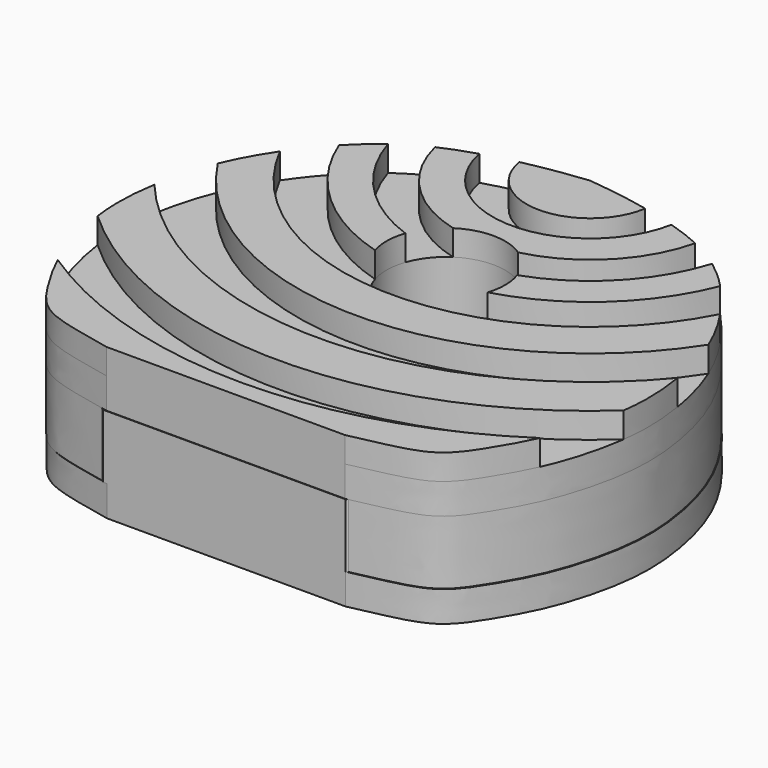
from build123d import *

# Parameters (mm, degrees)
F1_DEPTH  = 2.5
F2_R      = 2.2928226191
F3_DEPTH  = 25.4
F5_DEPTH  = 1.2
F8_DEPTH  = 2.5
F9_DEPTH  = 1.2
F10_R     = 2.3288193764
F11_DEPTH = 25.4
F13_DEPTH = 1


# Not quite as in the source:
# - after a boolean that leaves OpenCascade's solid faulty, fix() repairs it


with BuildPart() as f1:
    # F0 (on Top) → F1 (new body)
    with BuildSketch(Plane.XY):
        with BuildLine():
            ThreePointArc((-8.9879343286, 39.4452884793), (-13.7471402995, 56.3640609225), (-18.5063462704, 39.4452884793))
            Line((-18.5063462704, 39.4452884793), (-8.9879343286, 39.4452884793))
        make_face()
    extrude(amount=F1_DEPTH)

    # F2 (on Top) → F3 (cut)
    with BuildSketch(Plane.XY):
        with Locations((-13.6671839282, 50.2410940826)):
            Circle(F2_R)
    extrude(amount=F3_DEPTH, mode=Mode.SUBTRACT)

    # F4 (on Top) → F5 (join)
    with BuildSketch(Plane.XY):
        with BuildLine():
            add(Edge.make_bspline(
                [(-13.6700998992, 57.3167428374), (-12.2791459013, 57.1776458416), (-9.0720580617, 56.5741155476), (-6.3520616613, 54.8008037838), (-4.1044958722, 51.7145145132), (-3.3277388361, 48.8343071743), (-3.1695344368, 46.2953832393), (-3.9427728458, 43.353155853), (-4.9861142684, 41.5734784894), (-6.0248466508, 39.9837351848), (-7.6451300521, 39.7473392392), (-8.9879343286, 39.4452884793)],
                knots=[0, 0, 0, 0, 0.1391131435, 0.256793187, 0.3818563281, 0.493472527, 0.5970664143, 0.7096475295, 0.8035052556, 0.8866680838, 1, 1, 1, 1], degree=3))
            add(Edge.make_bspline(
                [(-13.6700998992, 57.3167428374), (-15.061053897, 57.1776458416), (-18.2681417367, 56.5741155476), (-20.988138137, 54.8008037838), (-23.2357039261, 51.7145145132), (-24.0124609622, 48.8343071743), (-24.1706653616, 46.2953832393), (-23.3974269525, 43.353155853), (-22.35408553, 41.5734784894), (-21.3153531475, 39.9837351848), (-19.6950697463, 39.7473392392), (-18.3522654697, 39.4452884793)],
                knots=[0, 0, 0, 0, 0.1391131435, 0.256793187, 0.3818563281, 0.493472527, 0.5970664143, 0.7096475295, 0.8035052556, 0.8866680838, 1, 1, 1, 1], degree=3))
            Line((-18.3522654697, 39.4452884793), (-8.9879343286, 39.4452884793))
        make_face()
    extrude(amount=-F5_DEPTH)

    # F7 (on offset) → F8 (join)
    with BuildSketch(Plane.XY.offset(2.5)):
        with BuildLine():
            add(Edge.make_bspline(
                [(-13.7050435878, 57.337269187), (-12.31408959, 57.1981721911), (-9.1070017503, 56.5946418971), (-6.38700535, 54.8213301333), (-4.1394395609, 51.7350408627), (-3.3626825248, 48.8548335238), (-3.2044781254, 46.3159095888), (-3.9777165345, 43.3736822025), (-5.021057957, 41.594004839), (-6.0597903395, 40.0042615343), (-7.6800737407, 39.7678655887), (-9.0228780173, 39.4658148289)],
                knots=[0, 0, 0, 0, 0.1391131435, 0.256793187, 0.3818563281, 0.493472527, 0.5970664143, 0.7096475295, 0.8035052556, 0.8866680838, 1, 1, 1, 1], degree=3))
            add(Edge.make_bspline(
                [(-13.7050435878, 57.337269187), (-15.0959975857, 57.1981721911), (-18.3030854253, 56.5946418971), (-21.0230818257, 54.8213301333), (-23.2706476148, 51.7350408627), (-24.0474046509, 48.8548335238), (-24.2056090503, 46.3159095888), (-23.4323706412, 43.3736822025), (-22.3890292186, 41.594004839), (-21.3502968362, 40.0042615343), (-19.7300134349, 39.7678655887), (-18.3872091584, 39.4658148289)],
                knots=[0, 0, 0, 0, 0.1391131435, 0.256793187, 0.3818563281, 0.493472527, 0.5970664143, 0.7096475295, 0.8035052556, 0.8866680838, 1, 1, 1, 1], degree=3))
            Line((-18.3872091584, 39.4658148289), (-9.0228780173, 39.4658148289))
        make_face()
    extrude(amount=-F8_DEPTH)

    # F7 (on offset) → F9 (join)
    with BuildSketch(Plane.XY.offset(2.5)):
        with BuildLine():
            add(Edge.make_bspline(
                [(-13.7050435878, 57.337269187), (-12.31408959, 57.1981721911), (-9.1070017503, 56.5946418971), (-6.38700535, 54.8213301333), (-4.1394395609, 51.7350408627), (-3.3626825248, 48.8548335238), (-3.2044781254, 46.3159095888), (-3.9777165345, 43.3736822025), (-5.021057957, 41.594004839), (-6.0597903395, 40.0042615343), (-7.6800737407, 39.7678655887), (-9.0228780173, 39.4658148289)],
                knots=[0, 0, 0, 0, 0.1391131435, 0.256793187, 0.3818563281, 0.493472527, 0.5970664143, 0.7096475295, 0.8035052556, 0.8866680838, 1, 1, 1, 1], degree=3))
            add(Edge.make_bspline(
                [(-13.7050435878, 57.337269187), (-15.0959975857, 57.1981721911), (-18.3030854253, 56.5946418971), (-21.0230818257, 54.8213301333), (-23.2706476148, 51.7350408627), (-24.0474046509, 48.8548335238), (-24.2056090503, 46.3159095888), (-23.4323706412, 43.3736822025), (-22.3890292186, 41.594004839), (-21.3502968362, 40.0042615343), (-19.7300134349, 39.7678655887), (-18.3872091584, 39.4658148289)],
                knots=[0, 0, 0, 0, 0.1391131435, 0.256793187, 0.3818563281, 0.493472527, 0.5970664143, 0.7096475295, 0.8035052556, 0.8866680838, 1, 1, 1, 1], degree=3))
            Line((-18.3872091584, 39.4658148289), (-9.0228780173, 39.4658148289))
        make_face()
    extrude(amount=F9_DEPTH)

    # F10 (on face) → F11 (cut)
    with BuildSketch(Plane.XY.offset(3.7)):
        with Locations((-13.7454718351, 50.3010265529)):
            Circle(F10_R)
    extrude(amount=-F11_DEPTH, mode=Mode.SUBTRACT)

    # F12 (on face) → F13 (join)
    with BuildSketch(Plane.XY.offset(3.7)):
        with BuildLine():
            add(Edge.make_bspline(
                [(-13.7050435878, 57.337269187), (-14.4653313277, 57.2612395406), (-15.3291200458, 57.1290853585), (-16.1737990809, 56.9432560968)],
                knots=[0, 0, 0, 0, 0.0760384726, 0.0760384726, 0.0760384726, 0.0760384726], degree=3))
            ThreePointArc((-16.1737990809, 56.9432560968), (-13.7050435878, 54.837269187), (-11.2362880947, 56.9432560968))
            add(Edge.make_bspline(
                [(-13.7050435878, 57.337269187), (-12.944755848, 57.2612395406), (-12.0809671299, 57.1290853585), (-11.2362880947, 56.9432560968)],
                knots=[0, 0, 0, 0, 0.0760384726, 0.0760384726, 0.0760384726, 0.0760384726], degree=3))
        make_face()
        with BuildLine():
            ThreePointArc((-9.9368932211, 56.6057620793), (-13.7050435878, 53.4987721067), (-17.4731939546, 56.6057620793))
            add(Edge.make_bspline(
                [(-17.4731939546, 56.6057620793), (-17.713095027, 56.5324460832), (-18.1815017641, 56.3748215542), (-18.6046452919, 56.1978491764), (-18.8084564971, 56.1028285931)],
                knots=[0.1160410133, 0.1160410133, 0.1160410133, 0.1160410133, 0.1391131435, 0.1625827971, 0.1625827971, 0.1625827971, 0.1625827971], degree=3))
            ThreePointArc((-18.8084564971, 56.1028285931), (-17.4454527537, 53.6524345673), (-15.0157350202, 52.2529054243))
            ThreePointArc((-15.0157350202, 52.2529054243), (-13.7320913228, 52.6298074893), (-12.452863378, 52.2381798934))
            ThreePointArc((-12.452863378, 52.2381798934), (-9.9858678234, 53.6310044183), (-8.6016306786, 56.1028285931))
            add(Edge.make_bspline(
                [(-9.9368932211, 56.6057620793), (-9.6969921487, 56.5324460832), (-9.2285854116, 56.3748215542), (-8.8054418837, 56.1978491764), (-8.6016306786, 56.1028285931)],
                knots=[0.1160410133, 0.1160410133, 0.1160410133, 0.1160410133, 0.1391131435, 0.1625827971, 0.1625827971, 0.1625827971, 0.1625827971], degree=3))
        make_face()
        with BuildLine():
            ThreePointArc((-15.9439411579, 51.0692272588), (-18.5092523241, 52.7306879861), (-20.0615521842, 55.3634884478))
            add(Edge.make_bspline(
                [(-20.0615521842, 55.3634884478), (-20.3622908826, 55.1424226516), (-20.7354717832, 54.8211081374), (-21.0991869423, 54.4504855004), (-21.184759468, 54.3600266085)],
                knots=[0.2154149552, 0.2154149552, 0.2154149552, 0.2154149552, 0.256793187, 0.2696740176, 0.2696740176, 0.2696740176, 0.2696740176], degree=3))
            ThreePointArc((-21.184759468, 54.3600266085), (-19.1249825347, 51.3845903924), (-15.9700219432, 49.6119862751))
            ThreePointArc((-15.9700219432, 49.6119862751), (-16.0739183221, 50.342699628), (-15.9439411579, 51.0692272588))
        make_face()
        with BuildLine():
            add(Edge.make_bspline(
                [(-7.3485349914, 55.3634884478), (-7.0477962931, 55.1424226516), (-6.6746153925, 54.8211081374), (-6.3109002333, 54.4504855004), (-6.2253277077, 54.3600266085)],
                knots=[0.2154149552, 0.2154149552, 0.2154149552, 0.2154149552, 0.256793187, 0.2696740176, 0.2696740176, 0.2696740176, 0.2696740176], degree=3))
            ThreePointArc((-7.3485349914, 55.3634884478), (-8.9273818183, 52.703160863), (-11.538320231, 51.0439138151))
            ThreePointArc((-11.538320231, 51.0439138151), (-11.4472706788, 50.6774188121), (-11.4166524587, 50.3010265529))
            ThreePointArc((-11.4166524587, 50.3010265529), (-11.4449073479, 49.9393599552), (-11.5289863986, 49.586469349))
            ThreePointArc((-11.5289863986, 49.586469349), (-8.319395937, 51.3535477363), (-6.2253277077, 54.3600266085))
        make_face()
        with BuildLine():
            ThreePointArc((-5.0678640605, 52.9127318674), (-13.7050435878, 47.632765043), (-22.3422231152, 52.9127318674))
            add(Edge.make_bspline(
                [(-22.3422231152, 52.9127318674), (-22.6243676708, 52.4958290759), (-22.9828123106, 51.88389324), (-23.2550467817, 51.2771618886), (-23.3282983496, 51.0995423986)],
                knots=[0.3317914228, 0.3317914228, 0.3317914228, 0.3317914228, 0.3818563281, 0.4026844082, 0.4026844082, 0.4026844082, 0.4026844082], degree=3))
            ThreePointArc((-23.3282983496, 51.0995423986), (-13.7050435878, 45.8692149625), (-4.0817888261, 51.0995423986))
            add(Edge.make_bspline(
                [(-5.0678640605, 52.9127318674), (-4.7857195048, 52.4958290759), (-4.427274865, 51.88389324), (-4.155040394, 51.2771618886), (-4.0817888261, 51.0995423986)],
                knots=[0.3317914228, 0.3317914228, 0.3317914228, 0.3317914228, 0.3818563281, 0.4026844082, 0.4026844082, 0.4026844082, 0.4026844082], degree=3))
        make_face()
        with BuildLine():
            ThreePointArc((-3.442200784, 48.7899550221), (-13.7050435878, 43.9812772041), (-23.9678863916, 48.7899550221))
            add(Edge.make_bspline(
                [(-23.9678863916, 48.7899550221), (-24.1027753964, 47.9656433641), (-24.1537367431, 47.107497335), (-24.0362338424, 46.1506221844), (-24.0261197487, 46.0757155585)],
                knots=[0.4950631574, 0.4950631574, 0.4950631574, 0.4950631574, 0.5970664143, 0.6056719545, 0.6056719545, 0.6056719545, 0.6056719545], degree=3))
            ThreePointArc((-24.0261197487, 46.0757155585), (-13.7050435878, 42.0615628777), (-3.3839674269, 46.0757155585))
            add(Edge.make_bspline(
                [(-3.442200784, 48.7899550221), (-3.3073117793, 47.9656433641), (-3.2563504326, 47.107497335), (-3.3738533332, 46.1506221844), (-3.3839674269, 46.0757155585)],
                knots=[0.4950631574, 0.4950631574, 0.4950631574, 0.4950631574, 0.5970664143, 0.6056719545, 0.6056719545, 0.6056719545, 0.6056719545], degree=3))
        make_face()
        with BuildLine():
            ThreePointArc((-4.2457875117, 43.0437652244), (-13.7050435878, 40.1972055627), (-23.164299664, 43.0437652244))
            add(Edge.make_bspline(
                [(-23.164299664, 43.0437652244), (-22.9110189824, 42.4853026214), (-22.3315365577, 41.5060143476), (-21.3502968362, 40.0042615343), (-19.7300134349, 39.7678655887), (-18.3872091584, 39.4658148289)],
                knots=[0.7257182099, 0.7257182099, 0.7257182099, 0.7257182099, 0.8035052556, 0.8866680838, 1, 1, 1, 1], degree=3))
            Line((-18.3872091584, 39.4658148289), (-9.0228780173, 39.4658148289))
            add(Edge.make_bspline(
                [(-4.2457875117, 43.0437652244), (-4.4990681933, 42.4853026214), (-5.0785506179, 41.5060143476), (-6.0597903395, 40.0042615343), (-7.6800737407, 39.7678655887), (-9.0228780173, 39.4658148289)],
                knots=[0.7257182099, 0.7257182099, 0.7257182099, 0.7257182099, 0.8035052556, 0.8866680838, 1, 1, 1, 1], degree=3))
        make_face()
    extrude(amount=F13_DEPTH)

    add(f1.part.fix(), mode=Mode.REPLACE)


solid = f1.part
